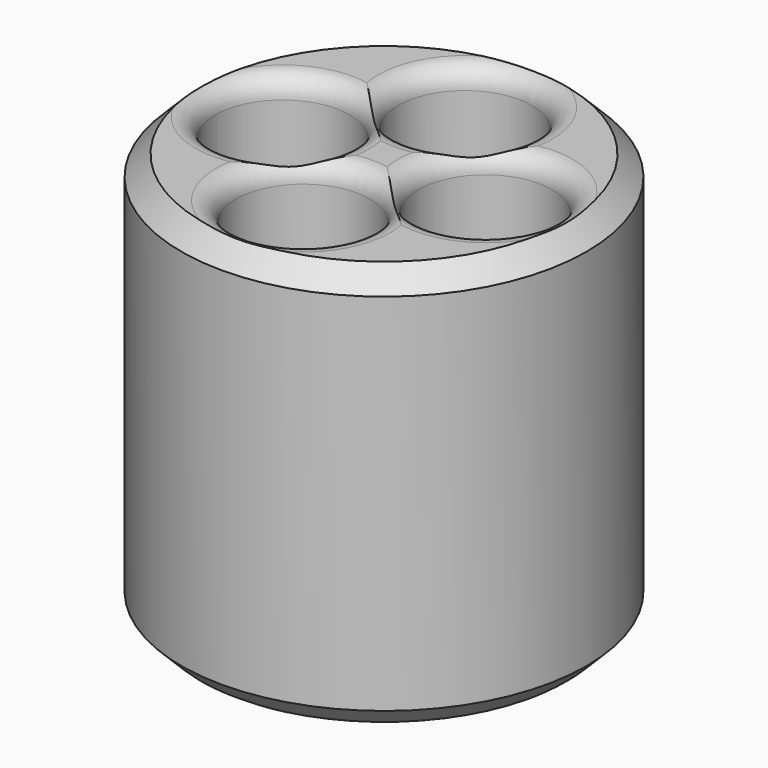
from build123d import *

# Parameters (mm, degrees)
F0_R     = 50
F0_R_2   = 16.5
F1_DEPTH = 100
F4_SIZE  = 5


# Not quite as in the source:
# - a fillet or chamfer that OpenCascade refuses, or shapes differently, is made with other operations: its cross-section is extruded or revolved along the edge and cut away or added


with BuildPart() as f1:
    # F0 (on Top) → F1 (new body)
    with BuildSketch(Plane.XY):
        Circle(F0_R)
        with Locations((0, -25)):
            Circle(F0_R_2, mode=Mode.SUBTRACT)
        with Locations((-25, 0)):
            Circle(F0_R_2, mode=Mode.SUBTRACT)
        with Locations((25, 0)):
            Circle(F0_R_2, mode=Mode.SUBTRACT)
        with Locations((0, 25)):
            Circle(F0_R_2, mode=Mode.SUBTRACT)
    extrude(amount=F1_DEPTH)

    # F2: fillet of radius 5 on 4 edges, made by hand

    # F2_s1 → F2_t2 (revolve, cut)
    with BuildSketch(Plane.XZ):
        with BuildLine():
            ThreePointArc((41.5, 95), (42.9644660941, 98.5355339059), (46.5, 100))
            Line((46.5, 100), (41.5, 100))
            Line((41.5, 100), (41.5, 95))
        make_face()
    revolve(axis=Axis((25, 0, 100), (0, 0, 1)), mode=Mode.SUBTRACT)

    # F2_s3 → F2_t4 (revolve, cut)
    with BuildSketch(Plane.XZ.offset(-25)):
        with BuildLine():
            ThreePointArc((16.5, 95), (17.9644660941, 98.5355339059), (21.5, 100))
            Line((21.5, 100), (16.5, 100))
            Line((16.5, 100), (16.5, 95))
        make_face()
    revolve(axis=Axis((0, 25, 100), (0, 0, 1)), mode=Mode.SUBTRACT)

    # F2_s5 → F2_t6 (revolve, cut)
    with BuildSketch(Plane.XZ):
        with BuildLine():
            ThreePointArc((-8.5, 95), (-7.0355339059, 98.5355339059), (-3.5, 100))
            Line((-3.5, 100), (-8.5, 100))
            Line((-8.5, 100), (-8.5, 95))
        make_face()
    revolve(axis=Axis((-25, 0, 100), (0, 0, 1)), mode=Mode.SUBTRACT)

    # F2_s7 → F2_t8 (revolve, cut)
    with BuildSketch(Plane.XZ.offset(25)):
        with BuildLine():
            ThreePointArc((16.5, 95), (17.9644660941, 98.5355339059), (21.5, 100))
            Line((21.5, 100), (16.5, 100))
            Line((16.5, 100), (16.5, 95))
        make_face()
    revolve(axis=Axis((0, -25, 100), (0, 0, 1)), mode=Mode.SUBTRACT)

    # F3: chamfer of 5 on 1 edges, made by hand

    # F3_s1 → F3_t2 (revolve, cut)
    with BuildSketch(Plane.XZ):
        Polygon((50, 95), (45, 100), (50, 100), align=None)
    revolve(axis=Axis((0, 0, 100), (0, 0, 1)), mode=Mode.SUBTRACT)

    # F4
    f4_edges = [f1.edges().sort_by_distance(p)[0] for p in [
        (-50, 0, 0),
    ]]
    chamfer(f4_edges, length=F4_SIZE)

    # F5: fillet of radius 5 on 4 edges, made by hand

    # F5_s1 → F5_t2 (revolve, cut)
    with BuildSketch(Plane.XZ):
        with BuildLine():
            ThreePointArc((-3.5, 0), (-7.0355339059, 1.4644660941), (-8.5, 5))
            Line((-8.5, 5), (-8.5, 0))
            Line((-8.5, 0), (-3.5, 0))
        make_face()
    revolve(axis=Axis((-25, 0, 0), (0, 0, 1)), mode=Mode.SUBTRACT)

    # F5_s3 → F5_t4 (revolve, cut)
    with BuildSketch(Plane.XZ.offset(-25)):
        with BuildLine():
            ThreePointArc((21.5, 0), (17.9644660941, 1.4644660941), (16.5, 5))
            Line((16.5, 5), (16.5, 0))
            Line((16.5, 0), (21.5, 0))
        make_face()
    revolve(axis=Axis((0, 25, 0), (0, 0, 1)), mode=Mode.SUBTRACT)

    # F5_s5 → F5_t6 (revolve, cut)
    with BuildSketch(Plane.XZ):
        with BuildLine():
            ThreePointArc((46.5, 0), (42.9644660941, 1.4644660941), (41.5, 5))
            Line((41.5, 5), (41.5, 0))
            Line((41.5, 0), (46.5, 0))
        make_face()
    revolve(axis=Axis((25, 0, 0), (0, 0, 1)), mode=Mode.SUBTRACT)

    # F5_s7 → F5_t8 (revolve, cut)
    with BuildSketch(Plane.XZ.offset(25)):
        with BuildLine():
            ThreePointArc((21.5, 0), (17.9644660941, 1.4644660941), (16.5, 5))
            Line((16.5, 5), (16.5, 0))
            Line((16.5, 0), (21.5, 0))
        make_face()
    revolve(axis=Axis((0, -25, 0), (0, 0, 1)), mode=Mode.SUBTRACT)


solid = f1.part
